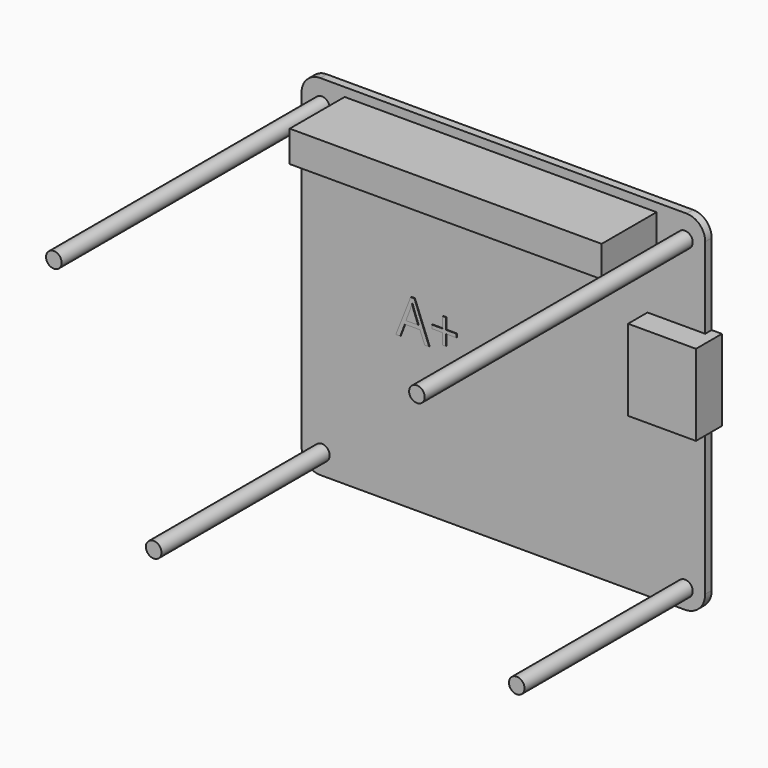
from build123d import *

# Parameters (mm, degrees)
F0_R          = 1.25
F0_W          = 50
F0_H          = 5
F1_DEPTH      = 1.3
F2_DEPTH      = 12.3
F0_W_2        = 9.25
F0_H_2        = 13
F0_W_3        = 1.64
F3_DEPTH      = 5.2
F0_TEXT_SIZE  = 8.4436246349
F4_DEPTH      = 1.4
F5_DEPTH      = 1.5
F6_DEPTH      = 55
F6_DEPTH_BACK = 2
F7_DEPTH      = 35
F7_DEPTH_BACK = 2


# Not quite as in the source:
# - Text() gives the source's letters only with a copy of the font that has no kerning and outlines rounded to 1/6400 em; it was checked with that copy


with BuildPart() as f1:
    # F0 (on Front) → F1 (new body)
    with BuildSketch(Plane.XZ):
        with BuildLine():
            Line((31.5453107178, 20.8069748506), (31.5453107178, 21.5584108519))
            ThreePointArc((31.5453107178, 21.5584108519), (30.6671388252, 23.67922331), (28.5467470628, 24.558410508))
            Line((28.5467470628, 24.558410508), (-30.153252937, 24.5865149939))
            ThreePointArc((-30.153252937, 24.5865149939), (-32.2755017401, 23.7083434452), (-33.154689282, 21.5865153378))
            Line((-33.154689282, 21.5865153378), (-33.1546892951, -28.4430251494))
            ThreePointArc((-33.1546892951, -28.4430251494), (-32.2760096387, -30.564345493), (-30.1546892951, -31.4430251494))
            Line((-30.1546892951, -31.4430251494), (28.2953107178, -31.4430251494))
            ThreePointArc((28.2953107178, -31.4430251494), (30.5934077567, -30.4911221883), (31.5453107178, -28.1930251494))
            Line((31.5453107178, -28.1930251494), (31.5453107178, -4.4430251494))
            Line((31.5453107178, -4.4430251494), (22.2953107178, -4.4430251494))
            Line((22.2953107178, -4.4430251494), (22.2953107178, 8.5569748506))
            Line((22.2953107178, 8.5569748506), (31.5453107178, 8.5569748506))
            Line((31.5453107178, 8.5569748506), (31.5453107178, 20.8069748506))
        make_face()
        with Locations((-29.9046892822, -28.1930251494)):
            Circle(F0_R, mode=Mode.SUBTRACT)
        Polygon((-12.6195598114, -7.5961076654), (-13.3451838034, -7.5961076654), (-14.0958748061, -5.6791410101), (-16.5115430415, -5.6791410101), (-17.2529988298, -7.5961076654), (-17.9627910256, -7.5961076654), (-15.580105699, -1.5430842553), (-14.9903712909, -1.5430842553), align=None, mode=Mode.SUBTRACT)
        Polygon((-9.9268351426, -2.5708316913), (-9.9268351426, -4.3347576502), (-8.2288750012, -4.3347576502), (-8.2288750012, -4.9033829967), (-9.9268351426, -4.9033829967), (-9.9268351426, -6.6607123739), (-10.5007377545, -6.6607123739), (-10.5007377545, -4.9033829967), (-12.1907819979, -4.9033829967), (-12.1907819979, -4.3347576502), (-10.5007377545, -4.3347576502), (-10.5007377545, -2.5708316913), align=None, mode=Mode.SUBTRACT)
        with Locations((28.2953107178, -28.4304671896)):
            Circle(F0_R, mode=Mode.SUBTRACT)
        with Locations((-29.9046892822, 20.8365149939)):
            Circle(F0_R, mode=Mode.SUBTRACT)
        with Locations((-1.2546892822, 20.6827428389)):
            Rectangle(F0_W, F0_H, mode=Mode.SUBTRACT)
        with Locations((28.2953107178, 20.8069748506)):
            Circle(F0_R, mode=Mode.SUBTRACT)
    extrude(amount=F1_DEPTH)

    # F0 (on Front) → F2 (join)
    with BuildSketch(Plane.XZ):
        with Locations((-1.2546892822, 20.6827428389)):
            Rectangle(F0_W, F0_H)
    extrude(amount=F2_DEPTH)

    # F0 (on Front) → F3 (join)
    with BuildSketch(Plane.XZ):
        with Locations((26.9203107178, 2.0569748506)):
            Rectangle(F0_W_2, F0_H_2)
        with Locations((32.3653107178, 2.0569748506)):
            Rectangle(F0_W_3, F0_H_2)
    extrude(amount=F3_DEPTH)

    # F0 (on Front) → F4 (join)
    with BuildSketch(Plane.XZ):
        with BuildLine():
            Line((-16.2635115679, -5.0485077951), (-14.3135620037, -5.0485077951))
            Line((-14.3135620037, -5.0485077951), (-15.0154383015, -3.1803558447))
            add(Edge.make_bspline(
                [(-15.0154383015, -3.1803558447), (-15.1513278855, -2.8254597467), (-15.2951333675, -2.3109263705)],
                knots=[0, 0, 0, 1, 1, 1], degree=2))
            add(Edge.make_bspline(
                [(-15.2951333675, -2.3109263705), (-15.3861661956, -2.7067212753), (-15.5550386883, -3.1803558447)],
                knots=[0, 0, 0, 1, 1, 1], degree=2))
            Line((-15.5550386883, -3.1803558447), (-16.2635115679, -5.0485077951))
        make_face()
        with Locations((-17.9627910256, -7.5961076654)):
            Text('A+', F0_TEXT_SIZE, font='Open Sans', text_align=(TextAlign.LEFT, TextAlign.BOTTOM))
    extrude(amount=F4_DEPTH)

    # F0 (on Front) → F5 (join)
    with BuildSketch(Plane.XZ):
        with BuildLine():
            Line((-16.2635115679, -5.0485077951), (-14.3135620037, -5.0485077951))
            Line((-14.3135620037, -5.0485077951), (-15.0154383015, -3.1803558447))
            add(Edge.make_bspline(
                [(-15.0154383015, -3.1803558447), (-15.1513278855, -2.8254597467), (-15.2951333675, -2.3109263705)],
                knots=[0, 0, 0, 1, 1, 1], degree=2))
            add(Edge.make_bspline(
                [(-15.2951333675, -2.3109263705), (-15.3861661956, -2.7067212753), (-15.5550386883, -3.1803558447)],
                knots=[0, 0, 0, 1, 1, 1], degree=2))
            Line((-15.5550386883, -3.1803558447), (-16.2635115679, -5.0485077951))
        make_face()
    extrude(amount=F5_DEPTH)

    # F0 (on Front) → F6 (join, two sides)
    with BuildSketch(Plane.XZ) as f6_sk:
        with Locations((28.2953107178, 20.8069748506)):
            Circle(F0_R)
        with Locations((-29.9046892822, 20.8365149939)):
            Circle(F0_R)
    extrude(amount=F6_DEPTH)
    extrude(f6_sk.sketch, amount=-F6_DEPTH_BACK)

    # F0 (on Front) → F7 (join, two sides)
    with BuildSketch(Plane.XZ) as f7_sk:
        with Locations((-29.9046892822, -28.1930251494)):
            Circle(F0_R)
        with Locations((28.2953107178, -28.4304671896)):
            Circle(F0_R)
    extrude(amount=F7_DEPTH)
    extrude(f7_sk.sketch, amount=-F7_DEPTH_BACK)


solid = f1.part
